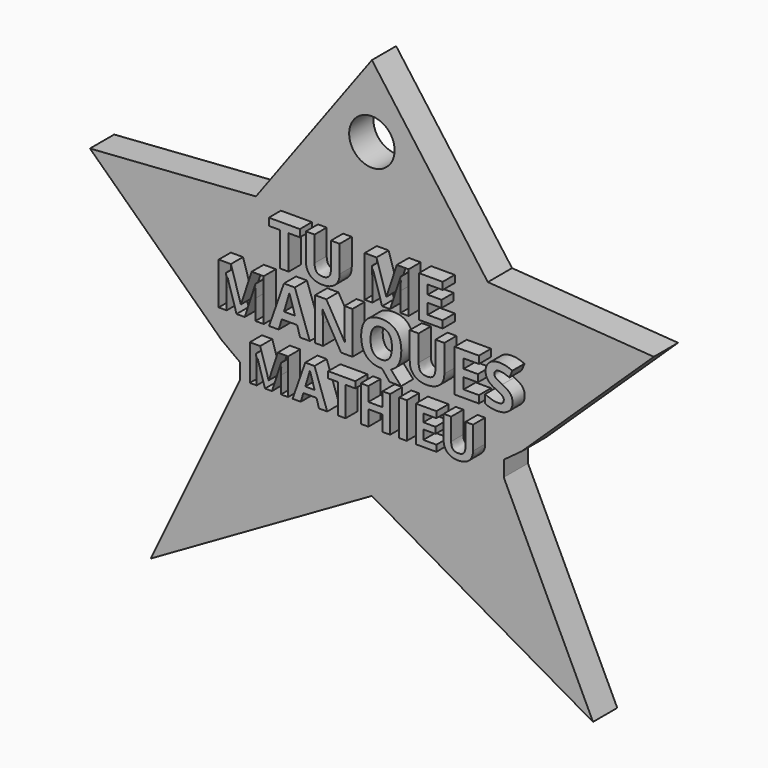
from build123d import *

# Parameters (mm, degrees)
F0_W           = 1.0027233238
F0_H           = 4.728011214
F0_R           = 3
F1_DEPTH       = 4
F0_TEXT_SIZE   = 6.6227340271
F0_TEXT_SIZE_2 = 7.7915753591
F0_TEXT_SIZE_3 = 7.6036633256
F2_DEPTH       = 6


# Not quite as in the source:
# - Text() gives the source's letters only with a copy of the font that has no kerning and outlines rounded to 1/6400 em; it was checked with that copy


with BuildPart() as f1:
    # F0 (on Front) → F1 (new body)
    with BuildSketch(Plane.XZ):
        Polygon((15.3086006659, 33.1815874028), (0, 54.0074984308), (-15.3086006659, 33.1815874028), (-37.2224335903, 31.6274128786), (-19.8157008339, 14.9977660316), (-17.4122109758, 13.2310214031), (-17.4122109758, 11.1680515805), (-29.1957038156, -13.4216465505), (-0.0016045015, 3.3528637946), (0, 3.3545432727), (0.0016045015, 3.3528637946), (29.1957038156, -13.4216465505), (17.4122109758, 11.1680515805), (17.4122109758, 13.2310214031), (19.8157008339, 14.9977660316), (37.2224335903, 31.6274128786), align=None)
        with BuildLine():
            Line((-11.5950636409, 12.5767774844), (-12.5139679872, 12.5767774844))
            Line((-12.5139679872, 12.5767774844), (-13.6522503981, 16.2855085396))
            Line((-13.6522503981, 16.2855085396), (-13.6812248594, 16.2855085396))
            add(Edge.make_bspline(
                [(-13.6812248594, 16.2855085396), (-13.6191367279, 15.154469744), (-13.6191367279, 14.7757321418)],
                knots=[0, 0, 0, 1, 1, 1], degree=2))
            Line((-13.6191367279, 14.7757321418), (-13.6191367279, 12.5767774844))
            Line((-13.6191367279, 12.5767774844), (-14.515275426, 12.5767774844))
            Line((-14.515275426, 12.5767774844), (-14.515275426, 17.3047886984))
            Line((-14.515275426, 17.3047886984), (-13.1503713351, 17.3047886984))
            Line((-13.1503713351, 17.3047886984), (-12.0317501658, 13.6891898405))
            Line((-12.0317501658, 13.6891898405), (-12.0120889242, 13.6891898405))
            Line((-12.0120889242, 13.6891898405), (-10.8251708103, 17.3047886984))
            Line((-10.8251708103, 17.3047886984), (-9.4613015216, 17.3047886984))
            Line((-9.4613015216, 17.3047886984), (-9.4613015216, 12.5767774844))
            Line((-9.4613015216, 12.5767774844), (-10.3957279007, 12.5767774844))
            Line((-10.3957279007, 12.5767774844), (-10.3957279007, 14.8150546251))
            add(Edge.make_bspline(
                [(-10.3957279007, 14.8150546251), (-10.3957279007, 14.9733793605), (-10.3905538898, 15.1803397988)],
                knots=[0, 0, 0, 1, 1, 1], degree=2))
            add(Edge.make_bspline(
                [(-10.3905538898, 15.1803397988), (-10.3853798788, 15.3873002372), (-10.3470921977, 16.2792997264)],
                knots=[0, 0, 0, 1, 1, 1], degree=2))
            Line((-10.3470921977, 16.2792997264), (-10.3760666591, 16.2792997264))
            Line((-10.3760666591, 16.2792997264), (-11.5950636409, 12.5767774844))
        make_face(mode=Mode.SUBTRACT)
        Polygon((-4.2966037827, 12.5767774844), (-5.3769372708, 12.5767774844), (-5.7194567963, 13.702642269), (-7.4434372477, 13.702642269), (-7.7859567732, 12.5767774844), (-8.8662902613, 12.5767774844), (-7.1971543261, 17.3244499401), (-5.9719485311, 17.3244499401), align=None, mode=Mode.SUBTRACT)
        Polygon((-1.8772362584, 16.4707381319), (-1.8772362584, 12.5767774844), (-2.8799595822, 12.5767774844), (-2.8799595822, 16.4707381319), (-4.1641491021, 16.4707381319), (-4.1641491021, 17.3047886984), (-0.5940815407, 17.3047886984), (-0.5940815407, 16.4707381319), align=None, mode=Mode.SUBTRACT)
        Polygon((4.0076838059, 17.3047886984), (4.0076838059, 12.5767774844), (3.0080648887, 12.5767774844), (3.0080648887, 14.6174074065), (1.1361077239, 14.6174074065), (1.1361077239, 12.5767774844), (0.1333844001, 12.5767774844), (0.1333844001, 17.3047886984), (1.1361077239, 17.3047886984), (1.1361077239, 15.451457973), (3.0080648887, 15.451457973), (3.0080648887, 17.3047886984), align=None, mode=Mode.SUBTRACT)
        with Locations((5.7021723949, 14.9407830914)):
            Rectangle(F0_W, F0_H, mode=Mode.SUBTRACT)
        Polygon((10.1161211437, 13.4046192378), (10.1161211437, 12.5767774844), (7.3935565773, 12.5767774844), (7.3935565773, 17.3047886984), (10.1161211437, 17.3047886984), (10.1161211437, 16.4831557582), (8.3962799011, 16.4831557582), (8.3962799011, 15.4452491599), (9.9971188917, 15.4452491599), (9.9971188917, 14.6236162197), (8.3962799011, 14.6236162197), (8.3962799011, 13.4046192378), align=None, mode=Mode.SUBTRACT)
        with BuildLine():
            Line((13.9510980662, 17.3047886984), (14.9507169835, 17.3047886984))
            Line((14.9507169835, 17.3047886984), (14.9507169835, 14.2459134197))
            add(Edge.make_bspline(
                [(14.9507169835, 14.2459134197), (14.9507169835, 13.7212687085), (14.716334287, 13.3270090734)],
                knots=[0, 0, 0, 1, 1, 1], degree=2))
            add(Edge.make_bspline(
                [(14.716334287, 13.3270090734), (14.4819515906, 12.9327494384), (14.0385388514, 12.7221671924)],
                knots=[0, 0, 0, 1, 1, 1], degree=2))
            add(Edge.make_bspline(
                [(14.0385388514, 12.7221671924), (13.5951261123, 12.5115849463), (12.9908016323, 12.5115849463)],
                knots=[0, 0, 0, 1, 1, 1], degree=2))
            add(Edge.make_bspline(
                [(12.9908016323, 12.5115849463), (12.0791409014, 12.5115849463), (11.5746748329, 12.979315537)],
                knots=[0, 0, 0, 1, 1, 1], degree=2))
            add(Edge.make_bspline(
                [(11.5746748329, 12.979315537), (11.0702087645, 13.4470461277), (11.0702087645, 14.258331046)],
                knots=[0, 0, 0, 1, 1, 1], degree=2))
            Line((11.0702087645, 14.258331046), (11.0702087645, 17.3047886984))
            Line((11.0702087645, 17.3047886984), (12.0687928795, 17.3047886984))
            Line((12.0687928795, 17.3047886984), (12.0687928795, 14.4104469682))
            add(Edge.make_bspline(
                [(12.0687928795, 14.4104469682), (12.0687928795, 13.8640714109), (12.2886883452, 13.6084752696)],
                knots=[0, 0, 0, 1, 1, 1], degree=2))
            add(Edge.make_bspline(
                [(12.2886883452, 13.6084752696), (12.508583811, 13.3528791282), (13.0166716871, 13.3528791282)],
                knots=[0, 0, 0, 1, 1, 1], degree=2))
            add(Edge.make_bspline(
                [(13.0166716871, 13.3528791282), (13.5082027282, 13.3528791282), (13.7296503972, 13.6100274729)],
                knots=[0, 0, 0, 1, 1, 1], degree=2))
            add(Edge.make_bspline(
                [(13.7296503972, 13.6100274729), (13.9510980662, 13.8671758175), (13.9510980662, 14.4166557813)],
                knots=[0, 0, 0, 1, 1, 1], degree=2))
            Line((13.9510980662, 14.4166557813), (13.9510980662, 17.3047886984))
        make_face(mode=Mode.SUBTRACT)
        with BuildLine():
            Line((-15.1862683527, 20.0173470582), (-16.2673494338, 20.0173470582))
            Line((-16.2673494338, 20.0173470582), (-17.6065264486, 24.3806292594))
            Line((-17.6065264486, 24.3806292594), (-17.6406145908, 24.3806292594))
            add(Edge.make_bspline(
                [(-17.6406145908, 24.3806292594), (-17.5675685718, 23.0499742801), (-17.5675685718, 22.6043935642)],
                knots=[0, 0, 0, 1, 1, 1], degree=2))
            Line((-17.5675685718, 22.6043935642), (-17.5675685718, 20.0173470582))
            Line((-17.5675685718, 20.0173470582), (-18.6218661126, 20.0173470582))
            Line((-18.6218661126, 20.0173470582), (-18.6218661126, 25.5798014045))
            Line((-18.6218661126, 25.5798014045), (-17.0160711284, 25.5798014045))
            Line((-17.0160711284, 25.5798014045), (-15.7000253529, 21.3260882318))
            Line((-15.7000253529, 21.3260882318), (-15.6768941136, 21.3260882318))
            Line((-15.6768941136, 21.3260882318), (-14.2804977172, 25.5798014045))
            Line((-14.2804977172, 25.5798014045), (-12.6759201667, 25.5798014045))
            Line((-12.6759201667, 25.5798014045), (-12.6759201667, 20.0173470582))
            Line((-12.6759201667, 20.0173470582), (-13.7752627525, 20.0173470582))
            Line((-13.7752627525, 20.0173470582), (-13.7752627525, 22.6506560429))
            add(Edge.make_bspline(
                [(-13.7752627525, 22.6506560429), (-13.7752627525, 22.8369233913), (-13.7691755842, 23.0804101213)],
                knots=[0, 0, 0, 1, 1, 1], degree=2))
            add(Edge.make_bspline(
                [(-13.7691755842, 23.0804101213), (-13.763088416, 23.3238968513), (-13.718043371, 24.3733246575)],
                knots=[0, 0, 0, 1, 1, 1], degree=2))
            Line((-13.718043371, 24.3733246575), (-13.7521315131, 24.3733246575))
            Line((-13.7521315131, 24.3733246575), (-15.1862683527, 20.0173470582))
        make_face(mode=Mode.SUBTRACT)
        Polygon((-6.5997088202, 20.0173470582), (-7.8707095506, 20.0173470582), (-8.2736800888, 21.3419148693), (-10.3019245494, 21.3419148693), (-10.7048950875, 20.0173470582), (-11.975895818, 20.0173470582), (-10.0121753408, 25.6029326438), (-8.5707338993, 25.6029326438), align=None, mode=Mode.SUBTRACT)
        with BuildLine():
            Line((-0.9654258886, 25.5798014045), (-0.9654258886, 20.0173470582))
            Line((-0.9654258886, 20.0173470582), (-2.4640867116, 20.0173470582))
            Line((-2.4640867116, 20.0173470582), (-4.8843448075, 24.2247977522))
            Line((-4.8843448075, 24.2247977522), (-4.9184329497, 24.2247977522))
            add(Edge.make_bspline(
                [(-4.9184329497, 24.2247977522), (-4.8453869307, 23.1108459625), (-4.8453869307, 22.6348294055)],
                knots=[0, 0, 0, 1, 1, 1], degree=2))
            Line((-4.8453869307, 22.6348294055), (-4.8453869307, 20.0173470582))
            Line((-4.8453869307, 20.0173470582), (-5.8996844715, 20.0173470582))
            Line((-5.8996844715, 20.0173470582), (-5.8996844715, 25.5798014045))
            Line((-5.8996844715, 25.5798014045), (-4.4119805514, 25.5798014045))
            Line((-4.4119805514, 25.5798014045), (-1.99659219, 21.4137434546))
            Line((-1.99659219, 21.4137434546), (-1.9698086497, 21.4137434546))
            add(Edge.make_bspline(
                [(-1.9698086497, 21.4137434546), (-2.0270280313, 22.4984768367), (-2.0270280313, 22.9464924198)],
                knots=[0, 0, 0, 1, 1, 1], degree=2))
            Line((-2.0270280313, 22.9464924198), (-2.0270280313, 25.5798014045))
            Line((-2.0270280313, 25.5798014045), (-0.9654258886, 25.5798014045))
        make_face(mode=Mode.SUBTRACT)
        Polygon((-9.3833469314, 31.645837729), (-9.3833469314, 27.1751213081), (-10.5345890818, 27.1751213081), (-10.5345890818, 31.645837729), (-12.0089869235, 31.645837729), (-12.0089869235, 32.6034240791), (-7.910137162, 32.6034240791), (-7.910137162, 31.645837729), align=None, mode=Mode.SUBTRACT)
        with BuildLine():
            Line((-3.8041589662, 32.6034240791), (-2.656481033, 32.6034240791))
            Line((-2.656481033, 32.6034240791), (-2.656481033, 29.0914820806))
            add(Edge.make_bspline(
                [(-2.656481033, 29.0914820806), (-2.656481033, 28.4891293765), (-2.9255794304, 28.0364737942)],
                knots=[0, 0, 0, 1, 1, 1], degree=2))
            add(Edge.make_bspline(
                [(-2.9255794304, 28.0364737942), (-3.1946778278, 27.5838182118), (-3.7037668489, 27.3420454795)],
                knots=[0, 0, 0, 1, 1, 1], degree=2))
            add(Edge.make_bspline(
                [(-3.7037668489, 27.3420454795), (-4.21285587, 27.1002727472), (-4.9066901484, 27.1002727472)],
                knots=[0, 0, 0, 1, 1, 1], degree=2))
            add(Edge.make_bspline(
                [(-4.9066901484, 27.1002727472), (-5.9533819281, 27.1002727472), (-6.5325672205, 27.6372814696)],
                knots=[0, 0, 0, 1, 1, 1], degree=2))
            add(Edge.make_bspline(
                [(-6.5325672205, 27.6372814696), (-7.1117525129, 28.174290192), (-7.1117525129, 29.1057389494)],
                knots=[0, 0, 0, 1, 1, 1], degree=2))
            Line((-7.1117525129, 29.1057389494), (-7.1117525129, 32.6034240791))
            Line((-7.1117525129, 32.6034240791), (-5.965262652, 32.6034240791))
            Line((-5.965262652, 32.6034240791), (-5.965262652, 29.2803855914))
            add(Edge.make_bspline(
                [(-5.965262652, 29.2803855914), (-5.965262652, 28.653083367), (-5.7127972682, 28.3596294855)],
                knots=[0, 0, 0, 1, 1, 1], degree=2))
            add(Edge.make_bspline(
                [(-5.7127972682, 28.3596294855), (-5.4603318843, 28.0661756041), (-4.8769883386, 28.0661756041)],
                knots=[0, 0, 0, 1, 1, 1], degree=2))
            add(Edge.make_bspline(
                [(-4.8769883386, 28.0661756041), (-4.3126539511, 28.0661756041), (-4.0584064587, 28.3614115941)],
                knots=[0, 0, 0, 1, 1, 1], degree=2))
            add(Edge.make_bspline(
                [(-4.0584064587, 28.3614115941), (-3.8041589662, 28.6566475842), (-3.8041589662, 29.2875140257)],
                knots=[0, 0, 0, 1, 1, 1], degree=2))
            Line((-3.8041589662, 29.2875140257), (-3.8041589662, 32.6034240791))
        make_face(mode=Mode.SUBTRACT)
        with BuildLine():
            add(Edge.make_bspline(
                [(4.8039921781, 24.9290831186), (5.4833201547, 24.19070961), (5.4833201547, 22.8064875501)],
                knots=[0, 0, 0, 1, 1, 1], degree=2))
            add(Edge.make_bspline(
                [(5.4833201547, 22.8064875501), (5.4833201547, 21.8240185946), (5.1351341309, 21.1605172555)],
                knots=[0, 0, 0, 1, 1, 1], degree=2))
            add(Edge.make_bspline(
                [(5.1351341309, 21.1605172555), (4.786948107, 20.4970159163), (4.1137072986, 20.1890052029)],
                knots=[0, 0, 0, 1, 1, 1], degree=2))
            Line((4.1137072986, 20.1890052029), (5.4528843135, 18.6927792472))
            Line((5.4528843135, 18.6927792472), (3.942049154, 18.6927792472))
            Line((3.942049154, 18.6927792472), (2.9230571891, 19.9406487383))
            Line((2.9230571891, 19.9406487383), (2.8354019663, 19.9406487383))
            add(Edge.make_bspline(
                [(2.8354019663, 19.9406487383), (1.5570966339, 19.9406487383), (0.8722902059, 20.6826745479)],
                knots=[0, 0, 0, 1, 1, 1], degree=2))
            add(Edge.make_bspline(
                [(0.8722902059, 20.6826745479), (0.1874837778, 21.4247003575), (0.1874837778, 22.813792152)],
                knots=[0, 0, 0, 1, 1, 1], degree=2))
            add(Edge.make_bspline(
                [(0.1874837778, 22.813792152), (0.1874837778, 24.2028839465), (0.8741163563, 24.9351702869)],
                knots=[0, 0, 0, 1, 1, 1], degree=2))
            add(Edge.make_bspline(
                [(0.8741163563, 24.9351702869), (1.5607489349, 25.6674566273), (2.8427065682, 25.6674566273)],
                knots=[0, 0, 0, 1, 1, 1], degree=2))
            add(Edge.make_bspline(
                [(2.8427065682, 25.6674566273), (4.1246642015, 25.6674566273), (4.8039921781, 24.9290831186)],
                knots=[0, 0, 0, 1, 1, 1], degree=2))
        make_face(mode=Mode.SUBTRACT)
        with BuildLine():
            Line((9.9878246592, 25.5798014045), (11.163865565, 25.5798014045))
            Line((11.163865565, 25.5798014045), (11.163865565, 21.9810675355))
            add(Edge.make_bspline(
                [(11.163865565, 21.9810675355), (11.163865565, 21.363828675), (10.8881168433, 20.8999864544)],
                knots=[0, 0, 0, 1, 1, 1], degree=2))
            add(Edge.make_bspline(
                [(10.8881168433, 20.8999864544), (10.6123681216, 20.4361442338), (10.0906978027, 20.188396486)],
                knots=[0, 0, 0, 1, 1, 1], degree=2))
            add(Edge.make_bspline(
                [(10.0906978027, 20.188396486), (9.5690274837, 19.9406487383), (8.8580462322, 19.9406487383)],
                knots=[0, 0, 0, 1, 1, 1], degree=2))
            add(Edge.make_bspline(
                [(8.8580462322, 19.9406487383), (7.7854871866, 19.9406487383), (7.1919882823, 20.490928748)],
                knots=[0, 0, 0, 1, 1, 1], degree=2))
            add(Edge.make_bspline(
                [(7.1919882823, 20.490928748), (6.598489378, 21.0412087578), (6.598489378, 21.9956767393)],
                knots=[0, 0, 0, 1, 1, 1], degree=2))
            Line((6.598489378, 21.9956767393), (6.598489378, 25.5798014045))
            Line((6.598489378, 25.5798014045), (7.7733128501, 25.5798014045))
            Line((7.7733128501, 25.5798014045), (7.7733128501, 22.1746394858))
            add(Edge.make_bspline(
                [(7.7733128501, 22.1746394858), (7.7733128501, 21.5318345187), (8.0320175007, 21.2311284072)],
                knots=[0, 0, 0, 1, 1, 1], degree=2))
            add(Edge.make_bspline(
                [(8.0320175007, 21.2311284072), (8.2907221513, 20.9304222956), (8.8884820734, 20.9304222956)],
                knots=[0, 0, 0, 1, 1, 1], degree=2))
            add(Edge.make_bspline(
                [(8.8884820734, 20.9304222956), (9.4667630571, 20.9304222956), (9.7272938582, 21.2329545576)],
                knots=[0, 0, 0, 1, 1, 1], degree=2))
            add(Edge.make_bspline(
                [(9.7272938582, 21.2329545576), (9.9878246592, 21.5354868196), (9.9878246592, 22.1819440877)],
                knots=[0, 0, 0, 1, 1, 1], degree=2))
            Line((9.9878246592, 22.1819440877), (9.9878246592, 25.5798014045))
        make_face(mode=Mode.SUBTRACT)
        Polygon((15.729241752, 20.9912939781), (15.729241752, 20.0173470582), (12.5261738192, 20.0173470582), (12.5261738192, 25.5798014045), (15.729241752, 25.5798014045), (15.729241752, 24.6131590865), (13.7058670259, 24.6131590865), (13.7058670259, 23.3920731357), (15.5892368823, 23.3920731357), (15.5892368823, 22.4254308177), (13.7058670259, 22.4254308177), (13.7058670259, 20.9912939781), align=None, mode=Mode.SUBTRACT)
        with BuildLine():
            add(Edge.make_bspline(
                [(19.8837340822, 22.4808240487), (20.172874574, 22.1064632014), (20.172874574, 21.5622703599)],
                knots=[0, 0, 0, 1, 1, 1], degree=2))
            add(Edge.make_bspline(
                [(20.172874574, 21.5622703599), (20.172874574, 20.8086789307), (19.630507883, 20.3746638345)],
                knots=[0, 0, 0, 1, 1, 1], degree=2))
            add(Edge.make_bspline(
                [(19.630507883, 20.3746638345), (19.088141192, 19.9406487383), (18.1227163076, 19.9406487383)],
                knots=[0, 0, 0, 1, 1, 1], degree=2))
            add(Edge.make_bspline(
                [(18.1227163076, 19.9406487383), (17.2315548759, 19.9406487383), (16.5473571647, 20.2766604257)],
                knots=[0, 0, 0, 1, 1, 1], degree=2))
            Line((16.5473571647, 20.2766604257), (16.5473571647, 21.3723507105))
            add(Edge.make_bspline(
                [(16.5473571647, 21.3723507105), (17.109811511, 21.120341945), (17.4999989957, 21.0180775184)],
                knots=[0, 0, 0, 1, 1, 1], degree=2))
            add(Edge.make_bspline(
                [(17.4999989957, 21.0180775184), (17.8901864805, 20.9158130918), (18.2140238314, 20.9158130918)],
                knots=[0, 0, 0, 1, 1, 1], degree=2))
            add(Edge.make_bspline(
                [(18.2140238314, 20.9158130918), (18.601167732, 20.9158130918), (18.8087401693, 21.0637312803)],
                knots=[0, 0, 0, 1, 1, 1], degree=2))
            add(Edge.make_bspline(
                [(18.8087401693, 21.0637312803), (19.0163126066, 21.2116494688), (19.0163126066, 21.5050509784)],
                knots=[0, 0, 0, 1, 1, 1], degree=2))
            add(Edge.make_bspline(
                [(19.0163126066, 21.5050509784), (19.0163126066, 21.6681870875), (18.9250050829, 21.7960176207)],
                knots=[0, 0, 0, 1, 1, 1], degree=2))
            add(Edge.make_bspline(
                [(18.9250050829, 21.7960176207), (18.8336975592, 21.9238481539), (18.6565609631, 22.0413305011)],
                knots=[0, 0, 0, 1, 1, 1], degree=2))
            add(Edge.make_bspline(
                [(18.6565609631, 22.0413305011), (18.4794243671, 22.1588128484), (17.9352315256, 22.4181262158)],
                knots=[0, 0, 0, 1, 1, 1], degree=2))
            add(Edge.make_bspline(
                [(17.9352315256, 22.4181262158), (17.4263442599, 22.6579606448), (17.1712919103, 22.8783161354)],
                knots=[0, 0, 0, 1, 1, 1], degree=2))
            add(Edge.make_bspline(
                [(17.1712919103, 22.8783161354), (16.9162395606, 23.0986716261), (16.7640603544, 23.3920731357)],
                knots=[0, 0, 0, 1, 1, 1], degree=2))
            add(Edge.make_bspline(
                [(16.7640603544, 23.3920731357), (16.6118811482, 23.6854746453), (16.6118811482, 24.0762708469)],
                knots=[0, 0, 0, 1, 1, 1], degree=2))
            add(Edge.make_bspline(
                [(16.6118811482, 24.0762708469), (16.6118811482, 24.8152530724), (17.1122463783, 25.237093832)],
                knots=[0, 0, 0, 1, 1, 1], degree=2))
            add(Edge.make_bspline(
                [(17.1122463783, 25.237093832), (17.6126116084, 25.6589345917), (18.4952510045, 25.6589345917)],
                knots=[0, 0, 0, 1, 1, 1], degree=2))
            add(Edge.make_bspline(
                [(18.4952510045, 25.6589345917), (18.9286573839, 25.6589345917), (19.3224971696, 25.5566701651)],
                knots=[0, 0, 0, 1, 1, 1], degree=2))
            add(Edge.make_bspline(
                [(19.3224971696, 25.5566701651), (19.7163369553, 25.4544057385), (20.1460910337, 25.2681383901)],
                knots=[0, 0, 0, 1, 1, 1], degree=2))
            Line((20.1460910337, 25.2681383901), (19.766251735, 24.3501934181))
            add(Edge.make_bspline(
                [(19.766251735, 24.3501934181), (19.3206710191, 24.5328084656), (19.0297043768, 24.6052457678)],
                knots=[0, 0, 0, 1, 1, 1], degree=2))
            add(Edge.make_bspline(
                [(19.0297043768, 24.6052457678), (18.7387377345, 24.6776830699), (18.4575105614, 24.6776830699)],
                knots=[0, 0, 0, 1, 1, 1], degree=2))
            add(Edge.make_bspline(
                [(18.4575105614, 24.6776830699), (18.1227163076, 24.6776830699), (17.9437535611, 24.5218515627)],
                knots=[0, 0, 0, 1, 1, 1], degree=2))
            add(Edge.make_bspline(
                [(17.9437535611, 24.5218515627), (17.7647908146, 24.3660200556), (17.7647908146, 24.1152287237)],
                knots=[0, 0, 0, 1, 1, 1], degree=2))
            add(Edge.make_bspline(
                [(17.7647908146, 24.1152287237), (17.7647908146, 23.9593972165), (17.8372281168, 23.8431323029)],
                knots=[0, 0, 0, 1, 1, 1], degree=2))
            add(Edge.make_bspline(
                [(17.8372281168, 23.8431323029), (17.9096654189, 23.7268673894), (18.0673230766, 23.6185157945)],
                knots=[0, 0, 0, 1, 1, 1], degree=2))
            add(Edge.make_bspline(
                [(18.0673230766, 23.6185157945), (18.2249807342, 23.5101641997), (18.8142186208, 23.2289370266)],
                knots=[0, 0, 0, 1, 1, 1], degree=2))
            add(Edge.make_bspline(
                [(18.8142186208, 23.2289370266), (19.5945935903, 22.8551848961), (19.8837340822, 22.4808240487)],
                knots=[0, 0, 0, 1, 1, 1], degree=2))
        make_face(mode=Mode.SUBTRACT)
        with BuildLine():
            Line((4.0014766664, 27.1751213081), (2.94646838, 27.1751213081))
            Line((2.94646838, 27.1751213081), (1.6395887459, 31.4331727704))
            Line((1.6395887459, 31.4331727704), (1.6063227189, 31.4331727704))
            add(Edge.make_bspline(
                [(1.6063227189, 31.4331727704), (1.6776070625, 30.1346096431), (1.6776070625, 29.6997751467)],
                knots=[0, 0, 0, 1, 1, 1], degree=2))
            Line((1.6776070625, 29.6997751467), (1.6776070625, 27.1751213081))
            Line((1.6776070625, 27.1751213081), (0.6487363688, 27.1751213081))
            Line((0.6487363688, 27.1751213081), (0.6487363688, 32.6034240791))
            Line((0.6487363688, 32.6034240791), (2.2158038573, 32.6034240791))
            Line((2.2158038573, 32.6034240791), (3.5001101159, 28.4522991323))
            Line((3.5001101159, 28.4522991323), (3.5226834914, 28.4522991323))
            Line((3.5226834914, 28.4522991323), (4.885402528, 32.6034240791))
            Line((4.885402528, 32.6034240791), (6.4512819441, 32.6034240791))
            Line((6.4512819441, 32.6034240791), (6.4512819441, 27.1751213081))
            Line((6.4512819441, 27.1751213081), (5.3784525718, 27.1751213081))
            Line((5.3784525718, 27.1751213081), (5.3784525718, 29.7449218977))
            add(Edge.make_bspline(
                [(5.3784525718, 29.7449218977), (5.3784525718, 29.926696974), (5.3843929337, 30.164311453)],
                knots=[0, 0, 0, 1, 1, 1], degree=2))
            add(Edge.make_bspline(
                [(5.3843929337, 30.164311453), (5.3903332957, 30.4019259319), (5.4342919743, 31.426044336)],
                knots=[0, 0, 0, 1, 1, 1], degree=2))
            Line((5.4342919743, 31.426044336), (5.4010259473, 31.426044336))
            Line((5.4010259473, 31.426044336), (4.0014766664, 27.1751213081))
        make_face(mode=Mode.SUBTRACT)
        Polygon((10.9433836682, 28.1255792238), (10.9433836682, 27.1751213081), (7.8175651979, 27.1751213081), (7.8175651979, 32.6034240791), (10.9433836682, 32.6034240791), (10.9433836682, 31.6600945978), (8.9688073483, 31.6600945978), (8.9688073483, 30.468457986), (10.8067553428, 30.468457986), (10.8067553428, 29.5251285047), (8.9688073483, 29.5251285047), (8.9688073483, 28.1255792238), align=None, mode=Mode.SUBTRACT)
        with Locations((0, 44.4884373466)):
            Circle(F0_R, mode=Mode.SUBTRACT)
    extrude(amount=F1_DEPTH)

    # F0 (on Front) → F2 (join)
    with BuildSketch(Plane.XZ):
        with Locations((-15.1102866862, 12.5767774844)):
            Text('MATHIEU', F0_TEXT_SIZE, font='Open Sans', font_style=FontStyle.BOLD, text_align=(TextAlign.LEFT, TextAlign.BOTTOM))
        with Locations((-19.3218904613, 20.0173470582)):
            Text('MANQUES', F0_TEXT_SIZE_2, font='Open Sans', font_style=FontStyle.BOLD, text_align=(TextAlign.LEFT, TextAlign.BOTTOM))
        with Locations((-12.16106019, 27.1751213081)):
            Text('TU ME', F0_TEXT_SIZE_3, font='Open Sans', font_style=FontStyle.BOLD, text_align=(TextAlign.LEFT, TextAlign.BOTTOM))
    extrude(amount=F2_DEPTH)


with BuildPart() as f1b:
    # F0 (on Front) → F1, piece 2 (new body)
    with BuildSketch(Plane.XZ):
        with BuildLine():
            add(Edge.make_bspline(
                [(1.7817131423, 24.211405982), (1.4243963661, 23.7378242922), (1.4243963661, 22.8064875501)],
                knots=[0, 0, 0, 1, 1, 1], degree=2))
            add(Edge.make_bspline(
                [(1.4243963661, 22.8064875501), (1.4243963661, 21.8739333743), (1.7780608414, 21.402177835)],
                knots=[0, 0, 0, 1, 1, 1], degree=2))
            add(Edge.make_bspline(
                [(1.7780608414, 21.402177835), (2.1317253167, 20.9304222956), (2.8354019663, 20.9304222956)],
                knots=[0, 0, 0, 1, 1, 1], degree=2))
            add(Edge.make_bspline(
                [(2.8354019663, 20.9304222956), (4.2464075665, 20.9304222956), (4.2464075665, 22.8064875501)],
                knots=[0, 0, 0, 1, 1, 1], degree=2))
            add(Edge.make_bspline(
                [(4.2464075665, 22.8064875501), (4.2464075665, 24.6849876718), (2.8427065682, 24.6849876718)],
                knots=[0, 0, 0, 1, 1, 1], degree=2))
            add(Edge.make_bspline(
                [(2.8427065682, 24.6849876718), (2.1390299186, 24.6849876718), (1.7817131423, 24.211405982)],
                knots=[0, 0, 0, 1, 1, 1], degree=2))
        make_face()
    extrude(amount=F1_DEPTH)


with BuildPart() as f1c:
    # F0 (on Front) → F1, piece 3 (new body)
    with BuildSketch(Plane.XZ):
        with BuildLine():
            Line((-7.1909455129, 14.5429016487), (-5.9595309048, 14.5429016487))
            add(Edge.make_bspline(
                [(-5.9595309048, 14.5429016487), (-6.4345051108, 16.0723392881), (-6.4945236379, 16.2730909133)],
                knots=[0, 0, 0, 1, 1, 1], degree=2))
            add(Edge.make_bspline(
                [(-6.4945236379, 16.2730909133), (-6.554542165, 16.4738425385), (-6.5804122198, 16.5897403839)],
                knots=[0, 0, 0, 1, 1, 1], degree=2))
            add(Edge.make_bspline(
                [(-6.5804122198, 16.5897403839), (-6.6869968456, 16.1758195073), (-7.1909455129, 14.5429016487)],
                knots=[0, 0, 0, 1, 1, 1], degree=2))
        make_face()
    extrude(amount=F1_DEPTH)


with BuildPart() as f1d:
    # F0 (on Front) → F1, piece 4 (new body)
    with BuildSketch(Plane.XZ):
        with BuildLine():
            Line((-10.0048707389, 22.330470993), (-8.5561246955, 22.330470993))
            add(Edge.make_bspline(
                [(-8.5561246955, 22.330470993), (-9.1149267408, 24.1298379275), (-9.1855378925, 24.3660200556)],
                knots=[0, 0, 0, 1, 1, 1], degree=2))
            add(Edge.make_bspline(
                [(-9.1855378925, 24.3660200556), (-9.2561490442, 24.6022021836), (-9.2865848854, 24.7385547524)],
                knots=[0, 0, 0, 1, 1, 1], degree=2))
            add(Edge.make_bspline(
                [(-9.2865848854, 24.7385547524), (-9.4119805514, 24.2515812925), (-10.0048707389, 22.330470993)],
                knots=[0, 0, 0, 1, 1, 1], degree=2))
        make_face()
    extrude(amount=F1_DEPTH)


solid = Compound([f1.part, f1b.part, f1c.part, f1d.part])
